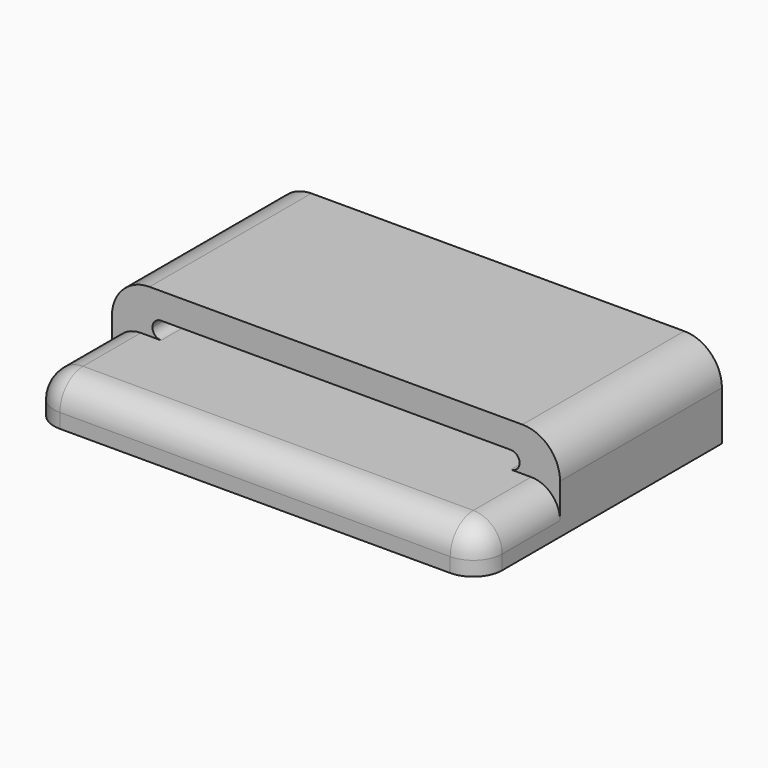
from build123d import *

# Parameters (mm, degrees)
F0_W         = 31
F0_H         = 21
F1_DEPTH     = 3
F2_W         = 31
F2_H         = 14
F3_DEPTH     = 3
F4_W         = 25.4
F4_H         = 1.2
F5_DEPTH     = 25
F6_W         = 25.4
F6_H         = 19.5
F7_DEPTH     = 1
F8_R         = 0.59999
F9_R         = 2.6
F10_W        = 25.4
F10_H        = 0.75
F11_DEPTH    = 0.5
F12_T4_DEPTH = 25.4
F12_T9_DEPTH = 25.4
F13_R        = 2
F14_SIZE     = 0.99999
F15_R        = 2


# Not quite as in the source:
# - a fillet or chamfer that OpenCascade refuses, or shapes differently, is made with other operations: its cross-section is extruded or revolved along the edge and cut away or added
# - a fillet or chamfer is up to 0.001 mm smaller than in the source, because OpenCascade refuses the exact size


with BuildPart() as f1:
    # F0 (on Top) → F1 (new body)
    with BuildSketch(Plane.XY):
        Rectangle(F0_W, F0_H)
    extrude(amount=F1_DEPTH)

    # F2 (on face) → F3 (join)
    with BuildSketch(Plane.XY.offset(3)):
        with Locations((0, 3.5)):
            Rectangle(F2_W, F2_H)
    extrude(amount=F3_DEPTH)

    # F4 (on face) → F5 (cut)
    with BuildSketch(Plane.XZ.offset(3.5)):
        with Locations((0, 3.6)):
            Rectangle(F4_W, F4_H)
    extrude(amount=-F5_DEPTH, mode=Mode.SUBTRACT)

    # F6 (on face) → F7 (cut)
    with BuildSketch(Plane(origin=(0, 0, 0), x_dir=(1, 0, 0), z_dir=(0, 0, -1))):
        with Locations((0, -0.75)):
            Rectangle(F6_W, F6_H)
    extrude(amount=-F7_DEPTH, mode=Mode.SUBTRACT)

    # F8 (radius 0.6 in the source; OpenCascade refuses exactly that, so slightly less here)
    f8_edges = [f1.edges().sort_by_distance(p)[0] for p in [
        (12.7, 3.5, 4.2),
        (12.7, 3.5, 3),
        (-12.7, 3.5, 3),
        (-12.7, 3.5, 4.2),
    ]]
    fillet(f8_edges, radius=F8_R)

    # F9
    f9_edges = [f1.edges().sort_by_distance(p)[0] for p in [
        (-15.5, 3.5, 6),
        (15.5, 3.5, 6),
    ]]
    fillet(f9_edges, radius=F9_R)

    # F10 (on face) → F11 (join)
    with BuildSketch(Plane(origin=(0, 0, 1), x_dir=(1, 0, 0), z_dir=(0, 0, -1))):
        with Locations((0, -0.375)):
            Rectangle(F10_W, F10_H)
    extrude(amount=F11_DEPTH)

    # F12: chamfer of 0.5 on 2 edges, made by hand


with BuildPart() as f12_tool2:
    # F12_s3 → F12_t4 (new body)
    with BuildSketch(Plane.YZ.offset(12.7)):
        Polygon((0.5, 0.5), (0, 1), (0, 0.5), align=None)
    extrude(amount=-F12_T4_DEPTH)

    split(bisect_by=Plane.XY.offset(1), keep=Keep.BOTTOM)


with BuildPart() as f1_1:
    add(f1.part)

    # F12_t1: cut F12_tool2
    add(f12_tool2.part, mode=Mode.SUBTRACT)


with BuildPart() as f12_tool7:
    # F12_s8 → F12_t9 (new body)
    with BuildSketch(Plane.YZ.offset(-12.7)):
        Polygon((0.75, 1), (0.25, 0.5), (0.75, 0.5), align=None)
    extrude(amount=F12_T9_DEPTH)

    split(bisect_by=Plane.XY.offset(1), keep=Keep.BOTTOM)


with BuildPart() as f1_2:
    add(f1_1.part)

    # F12_t6: cut F12_tool7
    add(f12_tool7.part, mode=Mode.SUBTRACT)

    # F13
    f13_edges = [f1_2.edges().sort_by_distance(p)[0] for p in [
        (15.5, -10.5, 1.5),
        (-15.5, -10.5, 1.5),
    ]]
    fillet(f13_edges, radius=F13_R)

    # F14 (size 1 in the source; OpenCascade refuses exactly that, so slightly less here)
    f14_edges = [f1_2.edges().sort_by_distance(p)[0] for p in [
        (0, -9, 1),
    ]]
    chamfer(f14_edges, length=F14_SIZE)

    # F15
    f15_edges = [f1_2.edges().sort_by_distance(p)[0] for p in [
        (0, -10.5, 3),
    ]]
    fillet(f15_edges, radius=F15_R)


solid = f1_2.part
